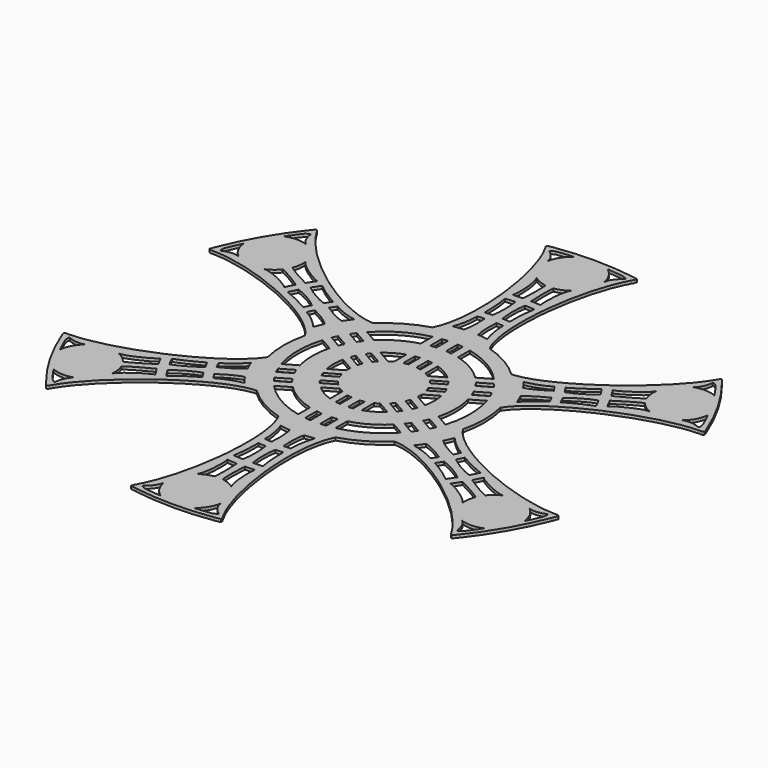
from build123d import *

# Parameters (mm, degrees)
F0_R     = 40.5
F1_DEPTH = 5
F2_COUNT = 6


with BuildPart() as f1:
    # F0 (on Top) → F1 (new body)
    with BuildSketch(Plane.XY):
        with BuildLine():
            ThreePointArc((-50, 167.7050983125), (-104.5825033168, -140.312152004), (175, 0))
            ThreePointArc((175, 0), (140.312152004, 104.5825033168), (50, 167.7050983125))
            ThreePointArc((50, 167.7050983125), (0, 175), (-50, 167.7050983125))
        make_face()
        with BuildLine():
            ThreePointArc((32.5, 146.4368464561), (116.993589568, 93.8749167776), (150, 0))
            ThreePointArc((150, 0), (-93.8749167776, -116.993589568), (-32.5, 146.4368464561))
            ThreePointArc((-32.5, 146.4368464561), (-25.4811216996, 147.8198648252), (-18.4042852942, 148.8666594064))
            ThreePointArc((-18.4042852942, 148.8666594064), (-13.4499363146, 149.3957804395), (-8.4807472475, 149.7600645236))
            ThreePointArc((-8.4807472475, 149.7600645236), (0, 150), (8.4807472475, 149.7600645236))
            ThreePointArc((8.4807472475, 149.7600645236), (13.4499363146, 149.3957804395), (18.4042852942, 148.8666594064))
            ThreePointArc((18.4042852942, 148.8666594064), (25.4811216996, 147.8198648252), (32.5, 146.4368464561))
        make_face(mode=Mode.SUBTRACT)
        with BuildLine():
            ThreePointArc((-50, 167.7050983125), (0, 175), (50, 167.7050983125))
            add(Edge.make_bspline(
                [(50, 167.7050983125), (47.3101972574, 172.6161198737), (45.0030030904, 178.4524809615), (43.0639425816, 185.0553885985)],
                knots=[0, 0, 0, 0, 26.2502119229, 26.2502119229, 26.2502119229, 26.2502119229], degree=3))
            ThreePointArc((43.0639425816, 185.0553885985), (36.5657089121, 186.4482473282), (30.0227383676, 187.6129931026))
            ThreePointArc((30.0227383676, 187.6129931026), (21.2828549204, 188.8042374695), (12.4971015407, 189.5885609763))
            ThreePointArc((12.4971015407, 189.5885609763), (0, 190), (-12.4971015407, 189.5885609763))
            ThreePointArc((-12.4971015407, 189.5885609763), (-21.2828549204, 188.8042374695), (-30.0227383676, 187.6129931026))
            ThreePointArc((-30.0227383676, 187.6129931026), (-36.5657089121, 186.4482473282), (-43.0639425816, 185.0553885985))
            add(Edge.make_bspline(
                [(-50, 167.7050983125), (-47.3101972574, 172.6161198737), (-45.0030030904, 178.4524809615), (-43.0639425816, 185.0553885985)],
                knots=[0, 0, 0, 0, 26.2502119229, 26.2502119229, 26.2502119229, 26.2502119229], degree=3))
        make_face()
        with BuildLine():
            ThreePointArc((30.0227383676, 187.6129931026), (36.5657089121, 186.4482473282), (43.0639425816, 185.0553885985))
            add(Edge.make_bspline(
                [(43.0639425816, 185.0553885985), (39.3930000751, 197.5557175983), (37.0414620924, 212.8033775266), (35.9111143264, 229.7209361732)],
                knots=[26.2502119229, 26.2502119229, 26.2502119229, 26.2502119229, 75.9459374111, 75.9459374111, 75.9459374111, 75.9459374111], degree=3))
            ThreePointArc((35.9111143264, 229.7209361732), (29.25660959, 230.6628870099), (22.5776601583, 231.4121127129))
            add(Edge.make_bspline(
                [(22.5776601583, 231.4121127129), (22.1983370871, 216.0993615618), (25.7666427642, 200.2952843904), (30.0227383676, 187.6129931026)],
                knots=[0, 0, 0, 0, 44.4273797132, 44.4273797132, 44.4273797132, 44.4273797132], degree=3))
        make_face()
        with BuildLine():
            add(Edge.make_bspline(
                [(-43.0639425816, 185.0553885985), (-39.3930000751, 197.5557175983), (-37.0414620924, 212.8033775266), (-35.9111143264, 229.7209361732)],
                knots=[26.2502119229, 26.2502119229, 26.2502119229, 26.2502119229, 75.9459374111, 75.9459374111, 75.9459374111, 75.9459374111], degree=3))
            ThreePointArc((-43.0639425816, 185.0553885985), (-36.5657089121, 186.4482473282), (-30.0227383676, 187.6129931026))
            add(Edge.make_bspline(
                [(-22.5776601583, 231.4121127129), (-22.1983370871, 216.0993615618), (-25.7666427642, 200.2952843904), (-30.0227383676, 187.6129931026)],
                knots=[0, 0, 0, 0, 44.4273797132, 44.4273797132, 44.4273797132, 44.4273797132], degree=3))
            ThreePointArc((-22.5776601583, 231.4121127129), (-29.25660959, 230.6628870099), (-35.9111143264, 229.7209361732))
        make_face()
        with BuildLine():
            ThreePointArc((22.5776601583, 231.4121127129), (29.25660959, 230.6628870099), (35.9111143264, 229.7209361732))
            add(Edge.make_bspline(
                [(35.9111143264, 229.7209361732), (35.5799986477, 234.6766401431), (35.3536726811, 239.7756372734), (35.2296676727, 244.9908448024)],
                knots=[75.9459374111, 75.9459374111, 75.9459374111, 75.9459374111, 90.5034341062, 90.5034341062, 90.5034341062, 90.5034341062], degree=3))
            ThreePointArc((35.2296676727, 244.9908448024), (28.5449735671, 245.8593663162), (21.8391068607, 246.5455270997))
            ThreePointArc((21.8391068607, 246.5455270997), (15.2483528522, 247.0407481705), (8.6467258396, 247.3598141445))
            ThreePointArc((8.6467258396, 247.3598141445), (0, 247.5108957629), (-8.6467258396, 247.3598141445))
            ThreePointArc((-8.6467258396, 247.3598141445), (-15.2483528522, 247.0407481705), (-21.8391068607, 246.5455270997))
            ThreePointArc((-21.8391068607, 246.5455270997), (-28.5449735671, 245.8593663162), (-35.2296676727, 244.9908448024))
            add(Edge.make_bspline(
                [(-35.9111143264, 229.7209361732), (-35.5799986477, 234.6766401431), (-35.3536726811, 239.7756372734), (-35.2296676727, 244.9908448024)],
                knots=[75.9459374111, 75.9459374111, 75.9459374111, 75.9459374111, 90.5034341062, 90.5034341062, 90.5034341062, 90.5034341062], degree=3))
            ThreePointArc((-35.9111143264, 229.7209361732), (-29.25660959, 230.6628870099), (-22.5776601583, 231.4121127129))
            ThreePointArc((-22.5776601583, 231.4121127129), (-16.4339311971, 231.9293913109), (-10.2786467879, 232.2835897533))
            ThreePointArc((-10.2786467879, 232.2835897533), (0, 232.5108957629), (10.2786467879, 232.2835897533))
            ThreePointArc((10.2786467879, 232.2835897533), (16.4339311971, 231.9293913109), (22.5776601583, 231.4121127129))
        make_face()
        with BuildLine():
            ThreePointArc((21.8391068607, 246.5455270997), (28.5449735671, 245.8593663162), (35.2296676727, 244.9908448024))
            add(Edge.make_bspline(
                [(35.2296676727, 244.9908448024), (34.8550578221, 260.7455964823), (35.4142278981, 277.5608829669), (36.8391170059, 294.6900615066)],
                knots=[90.5034341062, 90.5034341062, 90.5034341062, 90.5034341062, 134.4805422532, 134.4805422532, 134.4805422532, 134.4805422532], degree=3))
            ThreePointArc((36.8391170059, 294.6900615066), (31.1321580888, 295.3474930066), (25.4135504365, 295.8944141865))
            add(Edge.make_bspline(
                [(25.4135504365, 295.8944141865), (22.0925658941, 277.1417200565), (21.9646915793, 259.9910795689), (21.8391068607, 246.5455270997)],
                knots=[0, 0, 0, 0, 49.47816997, 49.47816997, 49.47816997, 49.47816997], degree=3))
        make_face()
        with BuildLine():
            ThreePointArc((-12.4971015407, 189.5885609763), (0, 190), (12.4971015407, 189.5885609763))
            add(Edge.make_bspline(
                [(10.2786467879, 232.2835897533), (9.2516251814, 218.6148708635), (9.126140736, 202.5039345026), (12.4971015407, 189.5885609763)],
                knots=[0, 0, 0, 0, 42.7526259282, 42.7526259282, 42.7526259282, 42.7526259282], degree=3))
            ThreePointArc((10.2786467879, 232.2835897533), (0, 232.5108957629), (-10.2786467879, 232.2835897533))
            add(Edge.make_bspline(
                [(-10.2786467879, 232.2835897533), (-9.2516251814, 218.6148708635), (-9.126140736, 202.5039345026), (-12.4971015407, 189.5885609763)],
                knots=[0, 0, 0, 0, 42.7526259282, 42.7526259282, 42.7526259282, 42.7526259282], degree=3))
        make_face()
        with BuildLine():
            add(Edge.make_bspline(
                [(-35.2296676727, 244.9908448024), (-34.8550578221, 260.7455964823), (-35.4142278981, 277.5608829669), (-36.8391170059, 294.6900615066)],
                knots=[90.5034341062, 90.5034341062, 90.5034341062, 90.5034341062, 134.4805422532, 134.4805422532, 134.4805422532, 134.4805422532], degree=3))
            ThreePointArc((-35.2296676727, 244.9908448024), (-28.5449735671, 245.8593663162), (-21.8391068607, 246.5455270997))
            add(Edge.make_bspline(
                [(-25.4135504365, 295.8944141865), (-22.0925658941, 277.1417200565), (-21.9646915793, 259.9910795689), (-21.8391068607, 246.5455270997)],
                knots=[0, 0, 0, 0, 49.47816997, 49.47816997, 49.47816997, 49.47816997], degree=3))
            ThreePointArc((-25.4135504365, 295.8944141865), (-31.1321580888, 295.3474930066), (-36.8391170059, 294.6900615066))
        make_face()
        with BuildLine():
            ThreePointArc((25.4135504365, 295.8944141865), (31.1321580888, 295.3474930066), (36.8391170059, 294.6900615066))
            add(Edge.make_bspline(
                [(36.8391170059, 294.6900615066), (37.2515484084, 299.6480691787), (37.7365099118, 304.6323747853), (38.2923510385, 309.6248722301)],
                knots=[134.4805422532, 134.4805422532, 134.4805422532, 134.4805422532, 147.2096313385, 147.2096313385, 147.2096313385, 147.2096313385], degree=3))
            ThreePointArc((38.2923510385, 309.6248722301), (31.315979306, 310.4080783286), (24.3237513157, 311.0341151281))
            ThreePointArc((24.3237513157, 311.0341151281), (15.7119026414, 311.5878716622), (7.0880327189, 311.9032308966))
            ThreePointArc((7.0880327189, 311.9032308966), (0, 311.9837586343), (-7.0880327189, 311.9032308966))
            ThreePointArc((-7.0880327189, 311.9032308966), (-15.7119026414, 311.5878716622), (-24.3237513157, 311.0341151281))
            ThreePointArc((-24.3237513157, 311.0341151281), (-31.315979306, 310.4080783286), (-38.2923510385, 309.6248722301))
            add(Edge.make_bspline(
                [(-36.8391170059, 294.6900615066), (-37.2515484084, 299.6480691787), (-37.7365099118, 304.6323747853), (-38.2923510385, 309.6248722301)],
                knots=[134.4805422532, 134.4805422532, 134.4805422532, 134.4805422532, 147.2096313385, 147.2096313385, 147.2096313385, 147.2096313385], degree=3))
            ThreePointArc((-36.8391170059, 294.6900615066), (-31.1321580888, 295.3474930066), (-25.4135504365, 295.8944141865))
            ThreePointArc((-25.4135504365, 295.8944141865), (-17.0518983945, 296.4938205995), (-8.6766595413, 296.8569831952))
            ThreePointArc((-8.6766595413, 296.8569831952), (0, 296.9837586343), (8.6766595413, 296.8569831952))
            ThreePointArc((8.6766595413, 296.8569831952), (17.0518983945, 296.4938205995), (25.4135504365, 295.8944141865))
        make_face()
        with BuildLine():
            ThreePointArc((24.3237513157, 311.0341151281), (31.315979306, 310.4080783286), (38.2923510385, 309.6248722301))
            add(Edge.make_bspline(
                [(38.2923510385, 309.6248722301), (43.9297576077, 360.2593728775), (56.8580242151, 411.7365070327), (75.3552994505, 445.167192013)],
                knots=[147.2096313385, 147.2096313385, 147.2096313385, 147.2096313385, 276.3095611136, 276.3095611136, 276.3095611136, 276.3095611136], degree=3))
            ThreePointArc((75.3552994505, 445.167192013), (73.3667030485, 445.4992445378), (71.3766437287, 445.8224138937))
            add(Edge.make_bspline(
                [(71.3766437287, 445.8224138937), (69.429333388, 444.8862411765), (67.4830520562, 443.7288841308), (65.5979515526, 442.3920762407)],
                knots=[0, 0, 0, 0, 6.5817479675, 6.5817479675, 6.5817479675, 6.5817479675], degree=3))
            add(Edge.make_bspline(
                [(65.5979515526, 442.3920762407), (57.2831650878, 436.4956945204), (50.1586569683, 427.1080809724), (49.38619588, 417.8104837562)],
                knots=[6.5817479675, 6.5817479675, 6.5817479675, 6.5817479675, 35.6124700999, 35.6124700999, 35.6124700999, 35.6124700999], degree=3))
            ThreePointArc((49.38619588, 417.8104837562), (49.8463127724, 413.9172826042), (50, 410))
            ThreePointArc((50, 410), (44.8418934092, 387.8820300325), (30.4318161807, 370.3275339317))
            add(Edge.make_bspline(
                [(30.4318161807, 370.3275339317), (22.9405183345, 360.9733319283), (21.3204508961, 316.4464912046), (24.3237513157, 311.0341151281)],
                knots=[0, 0, 0, 0, 59.6071972988, 59.6071972988, 59.6071972988, 59.6071972988], degree=3))
        make_face()
        with BuildLine():
            ThreePointArc((-8.6467258396, 247.3598141445), (0, 247.5108957629), (8.6467258396, 247.3598141445))
            add(Edge.make_bspline(
                [(8.6766595413, 296.8569831952), (5.9708249755, 283.543407917), (5.700296885, 262.9891205801), (8.6467258396, 247.3598141445)],
                knots=[0, 0, 0, 0, 49.497178102, 49.497178102, 49.497178102, 49.497178102], degree=3))
            ThreePointArc((8.6766595413, 296.8569831952), (0, 296.9837586343), (-8.6766595413, 296.8569831952))
            add(Edge.make_bspline(
                [(-8.6766595413, 296.8569831952), (-5.9708249755, 283.543407917), (-5.700296885, 262.9891205801), (-8.6467258396, 247.3598141445)],
                knots=[0, 0, 0, 0, 49.497178102, 49.497178102, 49.497178102, 49.497178102], degree=3))
        make_face()
        with BuildLine():
            add(Edge.make_bspline(
                [(-38.2923510385, 309.6248722301), (-43.9297576077, 360.2593728775), (-56.8580242151, 411.7365070327), (-75.3552994505, 445.167192013)],
                knots=[147.2096313385, 147.2096313385, 147.2096313385, 147.2096313385, 276.3095611136, 276.3095611136, 276.3095611136, 276.3095611136], degree=3))
            ThreePointArc((-38.2923510385, 309.6248722301), (-31.315979306, 310.4080783286), (-24.3237513157, 311.0341151281))
            add(Edge.make_bspline(
                [(-30.4318161807, 370.3275339317), (-22.9405183345, 360.9733319283), (-21.3204508961, 316.4464912046), (-24.3237513157, 311.0341151281)],
                knots=[0, 0, 0, 0, 59.6071972988, 59.6071972988, 59.6071972988, 59.6071972988], degree=3))
            ThreePointArc((-30.4318161807, 370.3275339317), (-46.4369076634, 391.463182402), (-49.38619588, 417.8104837562))
            add(Edge.make_bspline(
                [(-65.5979515526, 442.3920762407), (-57.2831650878, 436.4956945204), (-50.1586569683, 427.1080809724), (-49.38619588, 417.8104837562)],
                knots=[6.5817479675, 6.5817479675, 6.5817479675, 6.5817479675, 35.6124700999, 35.6124700999, 35.6124700999, 35.6124700999], degree=3))
            add(Edge.make_bspline(
                [(-71.3766437287, 445.8224138937), (-69.429333388, 444.8862411765), (-67.4830520562, 443.7288841308), (-65.5979515526, 442.3920762407)],
                knots=[0, 0, 0, 0, 6.5817479675, 6.5817479675, 6.5817479675, 6.5817479675], degree=3))
            ThreePointArc((-71.3766437287, 445.8224138937), (-73.3667030485, 445.4992445378), (-75.3552994505, 445.167192013))
        make_face()
        with BuildLine():
            ThreePointArc((71.3766437287, 445.8224138937), (73.3667030485, 445.4992445378), (75.3552994505, 445.167192013))
            add(Edge.make_bspline(
                [(75.3552994505, 445.167192013), (76.1612175197, 446.6237521144), (76.9777072727, 448.0460545293), (77.8046262978, 449.4325369727)],
                knots=[276.3095611136, 276.3095611136, 276.3095611136, 276.3095611136, 281.9343877338, 281.9343877338, 281.9343877338, 281.9343877338], degree=3))
            add(Edge.make_bspline(
                [(77.8046262978, 449.4325369727), (78.261457551, 451.2065528218), (78.3928268815, 452.4422361201), (78.2550810757, 453.2947631352)],
                knots=[0, 0, 0, 0, 2.3462542546, 2.3462542546, 2.3462542546, 2.3462542546], degree=3))
            ThreePointArc((78.2550810757, 453.2947631352), (73.1247545023, 454.1506030812), (67.9850790491, 454.9483806177))
            add(Edge.make_bspline(
                [(67.9850790491, 454.9483806177), (67.9185443898, 454.957823816), (67.8518848528, 454.9677638816), (67.785106852, 454.9782184776)],
                knots=[11.3381636187, 11.3381636187, 11.3381636187, 11.3381636187, 11.4518711693, 11.4518711693, 11.4518711693, 11.4518711693], degree=3))
            ThreePointArc((67.785106852, 454.9782184776), (33.9854344407, 458.7428367243), (1.172e-07, 460))
            ThreePointArc((1.172e-07, 460), (15.3691864442, 457.5792823406), (29.250194352, 450.5515243902))
            ThreePointArc((29.250194352, 450.5515243902), (43.8078404017, 449.3696953727), (58.3196436098, 447.7176221339))
            ThreePointArc((58.3196436098, 447.7176221339), (64.8550668099, 446.8177148559), (71.3766437287, 445.8224138937))
        make_face()
        with BuildLine():
            add(Edge.make_bspline(
                [(-75.3552994505, 445.167192013), (-76.1612175197, 446.6237521144), (-76.9777072727, 448.0460545293), (-77.8046262978, 449.4325369727)],
                knots=[276.3095611136, 276.3095611136, 276.3095611136, 276.3095611136, 281.9343877338, 281.9343877338, 281.9343877338, 281.9343877338], degree=3))
            ThreePointArc((-75.3552994505, 445.167192013), (-73.3667030485, 445.4992445378), (-71.3766437287, 445.8224138937))
            ThreePointArc((-71.3766437287, 445.8224138937), (-64.8550668099, 446.8177148559), (-58.3196436098, 447.7176221339))
            ThreePointArc((-58.3196436098, 447.7176221339), (-43.8078404017, 449.3696953727), (-29.250194352, 450.5515243902))
            ThreePointArc((-29.250194352, 450.5515243902), (-15.3691863327, 457.5792823766), (1.172e-07, 460))
            ThreePointArc((1.172e-07, 460), (-33.9854343238, 458.742836733), (-67.785106852, 454.9782184776))
            add(Edge.make_bspline(
                [(-67.9850790491, 454.9483806177), (-67.9185443898, 454.957823816), (-67.8518848528, 454.9677638816), (-67.785106852, 454.9782184776)],
                knots=[11.3381636187, 11.3381636187, 11.3381636187, 11.3381636187, 11.4518711693, 11.4518711693, 11.4518711693, 11.4518711693], degree=3))
            ThreePointArc((-67.9850790491, 454.9483806177), (-73.1247545023, 454.1506030812), (-78.2550810757, 453.2947631352))
            add(Edge.make_bspline(
                [(-77.8046262978, 449.4325369727), (-78.261457551, 451.2065528218), (-78.3928268815, 452.4422361201), (-78.2550810757, 453.2947631352)],
                knots=[0, 0, 0, 0, 2.3462542546, 2.3462542546, 2.3462542546, 2.3462542546], degree=3))
        make_face()
        with BuildLine():
            add(Edge.make_bspline(
                [(71.3766437287, 445.8224138937), (69.429333388, 444.8862411765), (67.4830520562, 443.7288841308), (65.5979515526, 442.3920762407)],
                knots=[0, 0, 0, 0, 6.5817479675, 6.5817479675, 6.5817479675, 6.5817479675], degree=3))
            ThreePointArc((71.3766437287, 445.8224138937), (64.8550668099, 446.8177148559), (58.3196436098, 447.7176221339))
            add(Edge.make_bspline(
                [(65.5979515526, 442.3920762407), (66.9932054286, 445.0014629003), (63.2680302576, 445.3519495123), (58.3196436098, 447.7176221339)],
                knots=[0, 0, 0, 0, 9.0186033049, 9.0186033049, 9.0186033049, 9.0186033049], degree=3))
        make_face()
        with BuildLine():
            ThreePointArc((-7.0880327189, 311.9032308966), (0, 311.9837586343), (7.0880327189, 311.9032308966))
            add(Edge.make_bspline(
                [(7.2053888568, 360.5219000827), (5.5626244284, 357.1719264984), (5.6422426887, 316.0084776703), (7.0880327189, 311.9032308966)],
                knots=[0, 0, 0, 0, 48.6188108235, 48.6188108235, 48.6188108235, 48.6188108235], degree=3))
            ThreePointArc((7.2053888568, 360.5219000827), (0, 360), (-7.2053888568, 360.5219000827))
            add(Edge.make_bspline(
                [(-7.2053888568, 360.5219000827), (-5.5626244284, 357.1719264984), (-5.6422426887, 316.0084776703), (-7.0880327189, 311.9032308966)],
                knots=[0, 0, 0, 0, 48.6188108235, 48.6188108235, 48.6188108235, 48.6188108235], degree=3))
        make_face()
        with BuildLine():
            ThreePointArc((7.2053888568, 360.5219000827), (19.44678417, 363.9367545059), (30.4318161807, 370.3275339317))
            ThreePointArc((30.4318161807, 370.3275339317), (44.8418934092, 387.8820300325), (50, 410))
            ThreePointArc((50, 410), (49.8463127724, 413.9172826042), (49.38619588, 417.8104837562))
            ThreePointArc((49.38619588, 417.8104837562), (42.5900739918, 436.1932357179), (29.250194352, 450.5515243902))
            ThreePointArc((29.250194352, 450.5515243902), (0, 451.5), (-29.250194352, 450.5515243902))
            ThreePointArc((-29.250194352, 450.5515243902), (-42.5900739918, 436.1932357179), (-49.38619588, 417.8104837562))
            ThreePointArc((-49.38619588, 417.8104837562), (-46.4369076634, 391.463182402), (-30.4318161807, 370.3275339317))
            ThreePointArc((-30.4318161807, 370.3275339317), (-19.44678417, 363.9367545059), (-7.2053888568, 360.5219000827))
            ThreePointArc((-7.2053888568, 360.5219000827), (0, 360), (7.2053888568, 360.5219000827))
        make_face()
        with Locations((0, 410)):
            Circle(F0_R, mode=Mode.SUBTRACT)
        with BuildLine():
            ThreePointArc((-58.3196436098, 447.7176221339), (-64.8550668099, 446.8177148559), (-71.3766437287, 445.8224138937))
            add(Edge.make_bspline(
                [(-71.3766437287, 445.8224138937), (-69.429333388, 444.8862411765), (-67.4830520562, 443.7288841308), (-65.5979515526, 442.3920762407)],
                knots=[0, 0, 0, 0, 6.5817479675, 6.5817479675, 6.5817479675, 6.5817479675], degree=3))
            add(Edge.make_bspline(
                [(-65.5979515526, 442.3920762407), (-66.9932054286, 445.0014629003), (-63.2680302576, 445.3519495123), (-58.3196436098, 447.7176221339)],
                knots=[0, 0, 0, 0, 9.0186033049, 9.0186033049, 9.0186033049, 9.0186033049], degree=3))
        make_face()
        with BuildLine():
            ThreePointArc((-29.250194352, 450.5515243902), (0, 451.5), (29.250194352, 450.5515243902))
            ThreePointArc((29.250194352, 450.5515243902), (15.3691864442, 457.5792823406), (1.172e-07, 460))
            ThreePointArc((1.172e-07, 460), (-15.3691863327, 457.5792823766), (-29.250194352, 450.5515243902))
        make_face()
        with BuildLine():
            Line((32.5, 120.7010770457), (32.5, 146.4368464561))
            ThreePointArc((32.5, 146.4368464561), (25.4811216996, 147.8198648252), (18.4042852942, 148.8666594064))
            Line((18.4042852942, 148.8666594064), (18.4042852942, 123.6377057487))
            ThreePointArc((18.4042852942, 123.6377057487), (25.494460425, 122.372515246), (32.5, 120.7010770457))
        make_face()
        with BuildLine():
            ThreePointArc((-18.4042852942, 148.8666594064), (-25.4811216996, 147.8198648252), (-32.5, 146.4368464561))
            Line((-32.5, 146.4368464561), (-32.5, 120.7010770457))
            ThreePointArc((-32.5, 120.7010770457), (-25.494460425, 122.372515246), (-18.4042852942, 123.6377057487))
            Line((-18.4042852942, 123.6377057487), (-18.4042852942, 148.8666594064))
        make_face()
        with BuildLine():
            ThreePointArc((125, 0), (99.2156741649, 76.0345316287), (32.5, 120.7010770457))
            ThreePointArc((32.5, 120.7010770457), (25.494460425, 122.372515246), (18.4042852942, 123.6377057487))
            ThreePointArc((18.4042852942, 123.6377057487), (13.4532433921, 124.2739322715), (8.4807472475, 124.7119758729))
            ThreePointArc((8.4807472475, 124.7119758729), (0, 125), (-8.4807472475, 124.7119758729))
            ThreePointArc((-8.4807472475, 124.7119758729), (-13.4532433921, 124.2739322715), (-18.4042852942, 123.6377057487))
            ThreePointArc((-18.4042852942, 123.6377057487), (-25.494460425, 122.372515246), (-32.5, 120.7010770457))
            ThreePointArc((-32.5, 120.7010770457), (-76.0345316287, -99.2156741649), (125, 0))
        make_face()
        with BuildLine():
            ThreePointArc((27.5, 83.0662386292), (70.9313047956, 51.2347538298), (87.5, 0))
            ThreePointArc((87.5, 0), (-51.2347538298, -70.9313047956), (-27.5, 83.0662386292))
            ThreePointArc((-27.5, 83.0662386292), (-21.3691268812, 84.8505180676), (-15.1244583415, 86.182949357))
            ThreePointArc((-15.1244583415, 86.182949357), (-11.094126399, 86.7938382574), (-7.0397162923, 87.2163539396))
            ThreePointArc((-7.0397162923, 87.2163539396), (0, 87.5), (7.0397162923, 87.2163539396))
            ThreePointArc((7.0397162923, 87.2163539396), (11.094126399, 86.7938382574), (15.1244583415, 86.182949357))
            ThreePointArc((15.1244583415, 86.182949357), (21.3691268812, 84.8505180676), (27.5, 83.0662386292))
        make_face(mode=Mode.SUBTRACT)
        with BuildLine():
            Line((8.4807472475, 124.7119758729), (8.4807472475, 149.7600645236))
            ThreePointArc((8.4807472475, 149.7600645236), (0, 150), (-8.4807472475, 149.7600645236))
            Line((-8.4807472475, 149.7600645236), (-8.4807472475, 124.7119758729))
            ThreePointArc((-8.4807472475, 124.7119758729), (0, 125), (8.4807472475, 124.7119758729))
        make_face()
        with BuildLine():
            Line((27.5, 56.1248608016), (27.5, 83.0662386292))
            ThreePointArc((27.5, 83.0662386292), (21.3691268812, 84.8505180676), (15.1244583415, 86.182949357))
            Line((15.1244583415, 86.182949357), (15.1244583415, 60.6424006771))
            ThreePointArc((15.1244583415, 60.6424006771), (21.4315924247, 58.7106195346), (27.5, 56.1248608016))
        make_face()
        with BuildLine():
            ThreePointArc((-15.1244583415, 86.182949357), (-21.3691268812, 84.8505180676), (-27.5, 83.0662386292))
            Line((-27.5, 83.0662386292), (-27.5, 56.1248608016))
            ThreePointArc((-27.5, 56.1248608016), (-21.4315924247, 58.7106195346), (-15.1244583415, 60.6424006771))
            Line((-15.1244583415, 60.6424006771), (-15.1244583415, 86.182949357))
        make_face()
        with BuildLine():
            ThreePointArc((62.5, 0), (53.033008589, 33.0718913883), (27.5, 56.1248608016))
            ThreePointArc((27.5, 56.1248608016), (21.4315924247, 58.7106195346), (15.1244583415, 60.6424006771))
            ThreePointArc((15.1244583415, 60.6424006771), (11.1061004221, 61.5053211797), (7.0397162923, 62.1022736663))
            ThreePointArc((7.0397162923, 62.1022736663), (0, 62.5), (-7.0397162923, 62.1022736663))
            ThreePointArc((-7.0397162923, 62.1022736663), (-11.1061004221, 61.5053211797), (-15.1244583415, 60.6424006771))
            ThreePointArc((-15.1244583415, 60.6424006771), (-21.4315924247, 58.7106195346), (-27.5, 56.1248608016))
            ThreePointArc((-27.5, 56.1248608016), (-33.0718913883, -53.033008589), (62.5, 0))
        make_face()
        with BuildLine():
            Line((7.0397162923, 62.1022736663), (7.0397162923, 87.2163539396))
            ThreePointArc((7.0397162923, 87.2163539396), (0, 87.5), (-7.0397162923, 87.2163539396))
            Line((-7.0397162923, 87.2163539396), (-7.0397162923, 62.1022736663))
            ThreePointArc((-7.0397162923, 62.1022736663), (0, 62.5), (7.0397162923, 62.1022736663))
        make_face()
        with Locations((0, 410)):
            Circle(F0_R)
    extrude(amount=F1_DEPTH)

    # F2: F1 ×6 about axis
    f2_axis = Axis((0, 0, 0), (0, 0, -1))


with BuildPart() as f1_1:
    add(f1.part)
    for i in range(1, F2_COUNT):
        add(f1.part.rotate(f2_axis, i * 360 / F2_COUNT))


solid = f1_1.part
